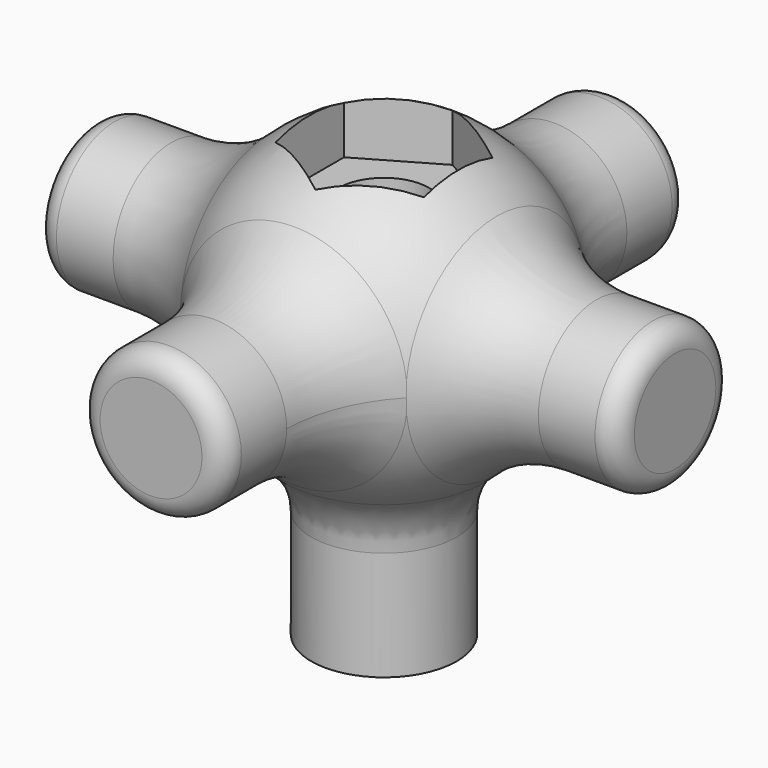
from build123d import *

# Parameters (mm, degrees)
F2_R          = 5
F3_DEPTH      = 20
F4_R          = 5
F5_DEPTH      = 20
F6_R          = 5
F7_DEPTH      = 20
F8_W          = 8.7868496776
F8_H          = 12.2011639178
F9_DEPTH      = 25
F11_DEPTH     = 19
F12_R         = 3.1
F13_DEPTH     = 43.50571
F15_R         = 5
F16_T2_ANGLE  = 180
F16_T4_ANGLE  = 180
F16_T6_ANGLE  = 180
F16_T8_ANGLE  = 180
F16_T10_ANGLE = 179.9999999891
F16_T12_ANGLE = 180.0000000129
F17_R         = 1.5
F18_R         = 1.5


# Not quite as in the source:
# - a fillet or chamfer that OpenCascade refuses, or shapes differently, is made with other operations: its cross-section is extruded or revolved along the edge and cut away or added


with BuildPart() as f1:
    # F0 (on Top) → F1 (revolve)
    with BuildSketch(Plane.XY):
        with BuildLine():
            ThreePointArc((-11, 0), (0, -11), (11, 0))
            Line((11, 0), (-11, 0))
        make_face()
    revolve(axis=Axis((0.2873940393, 0, 0), (1, 0, 0)))

    # F2 (on Top) → F3 (join)
    with BuildSketch(Plane.XY):
        Circle(F2_R)
    extrude(amount=-F3_DEPTH)

    # F4 (on Front) → F5 (join, symmetric)
    with BuildSketch(Plane.XZ):
        Circle(F4_R)
    extrude(amount=F5_DEPTH, both=True)

    # F6 (on Right) → F7 (join, symmetric)
    with BuildSketch(Plane.YZ):
        Circle(F6_R)
    extrude(amount=F7_DEPTH, both=True)

    # F10 (on face) → F11 (cut)
    with BuildSketch(Plane.XY.offset(25)):
        Polygon((-5.1, 2.9444863729), (-5.1, -2.9444863729), (0, -5.8889727457), (5.1, -2.9444863729), (5.1, 2.9444863729), (0, 5.8889727457), align=None)
    extrude(amount=-F11_DEPTH, mode=Mode.SUBTRACT)

    # F12 (on face) → F13 (cut)
    with BuildSketch(Plane.XY.offset(6)):
        Circle(F12_R)
    extrude(amount=-F13_DEPTH, mode=Mode.SUBTRACT)

    # F15
    f15_edges = [f1.edges().sort_by_distance(p)[0] for p in [
        (-5, 0, -9.797959),
    ]]
    fillet(f15_edges, radius=F15_R)

    # F16: fillet of radius 10 on 7 edges, made by hand

    # F16_s1 → F16_t2 (revolve)
    with BuildSketch(Plane.XY):
        with BuildLine():
            ThreePointArc((7.6978109292, -7.8571564232), (10.9173830992, -5.7415035459), (14.6977549306, -4.9996))
            Line((14.6977549306, -4.9996), (14.6977549306, -3.99936))
            ThreePointArc((14.6977549306, -3.99936), (12.2478569509, -3.99976), (9.7979589711, -3.99976))
            Line((9.7979589711, -3.99976), (8.9070216547, -4.5453454545))
            ThreePointArc((8.9070216547, -4.5453454545), (8.0579387192, -5.9215558476), (6.997816529, -7.1426720655))
            Line((6.997816529, -7.1426720655), (7.6978109292, -7.8571564232))
        make_face()
    revolve(axis=Axis((9.7979589711, 0, 0), (1, 0, 0)), revolution_arc=F16_T2_ANGLE)

    # F16_s3 → F16_t4 (revolve)
    with BuildSketch(Plane.XY):
        with BuildLine():
            ThreePointArc((7.6978109292, 7.8571564232), (10.9173830992, 5.7415035459), (14.6977549306, 4.9996))
            Line((14.6977549306, 4.9996), (14.6977549306, 3.99936))
            ThreePointArc((14.6977549306, 3.99936), (12.2478569509, 3.99976), (9.7979589711, 3.99976))
            Line((9.7979589711, 3.99976), (8.9070216547, 4.5453454545))
            ThreePointArc((8.9070216547, 4.5453454545), (8.0579387192, 5.9215558476), (6.997816529, 7.1426720655))
            Line((6.997816529, 7.1426720655), (7.6978109292, 7.8571564232))
        make_face()
    revolve(axis=Axis((9.7979589711, 0, 0), (1, 0, 0)), revolution_arc=F16_T4_ANGLE)

    # F16_s5 → F16_t6 (revolve)
    with BuildSketch(Plane.XY):
        with BuildLine():
            ThreePointArc((-7.6978109292, 7.8571564232), (-10.9173830992, 5.7415035459), (-14.6977549306, 4.9996))
            Line((-14.6977549306, 4.9996), (-14.6977549306, 3.99936))
            ThreePointArc((-14.6977549306, 3.99936), (-12.2478569509, 3.99976), (-9.7979589711, 3.99976))
            Line((-9.7979589711, 3.99976), (-8.9070216547, 4.5453454545))
            ThreePointArc((-8.9070216547, 4.5453454545), (-8.0579387192, 5.9215558476), (-6.997816529, 7.1426720655))
            Line((-6.997816529, 7.1426720655), (-7.6978109292, 7.8571564232))
        make_face()
    revolve(axis=Axis((-9.7979589711, 0, 0), (1, 0, 0)), revolution_arc=F16_T6_ANGLE)

    # F16_s7 → F16_t8 (revolve)
    with BuildSketch(Plane.XY):
        with BuildLine():
            ThreePointArc((-7.6978109292, -7.8571564232), (-10.9173830992, -5.7415035459), (-14.6977549306, -4.9996))
            Line((-14.6977549306, -4.9996), (-14.6977549306, -3.99936))
            ThreePointArc((-14.6977549306, -3.99936), (-12.2478569509, -3.99976), (-9.7979589711, -3.99976))
            Line((-9.7979589711, -3.99976), (-8.9070216547, -4.5453454545))
            ThreePointArc((-8.9070216547, -4.5453454545), (-8.0579387192, -5.9215558476), (-6.997816529, -7.1426720655))
            Line((-6.997816529, -7.1426720655), (-7.6978109292, -7.8571564232))
        make_face()
    revolve(axis=Axis((-9.7979589711, 0, 0), (1, 0, 0)), revolution_arc=F16_T8_ANGLE)

    # F16_s9 → F16_t10 (revolve)
    with BuildSketch(Plane.XY):
        with BuildLine():
            ThreePointArc((7.857156424, -7.6978109292), (5.7415035468, -10.9173830992), (4.9996000008, -14.6977549306))
            Line((4.9996000008, -14.6977549306), (3.9993600008, -14.6977549306))
            ThreePointArc((3.9993600008, -14.6977549306), (3.9997600008, -12.2478569509), (3.99976, -9.7979589711))
            Line((3.99976, -9.7979589711), (4.5453454546, -8.9070216546))
            ThreePointArc((4.5453454546, -8.9070216546), (5.9215558482, -8.0579387193), (7.1426720664, -6.997816529))
            Line((7.1426720664, -6.997816529), (7.857156424, -7.6978109292))
        make_face()
    revolve(axis=Axis((4e-10, -9.7979589711, -5e-10), (0, -1, 0)), revolution_arc=F16_T10_ANGLE)

    # F16_s11 → F16_t12 (revolve)
    with BuildSketch(Plane.XY):
        with BuildLine():
            ThreePointArc((-7.8571564226, -7.6978109292), (-5.7415035453, -10.9173830992), (-4.9995999994, -14.6977549306))
            Line((-4.9995999994, -14.6977549306), (-3.9993599994, -14.6977549306))
            ThreePointArc((-3.9993599994, -14.6977549306), (-3.9997599994, -12.2478569509), (-3.99976, -9.7979589711))
            Line((-3.99976, -9.7979589711), (-4.5453454545, -8.9070216547))
            ThreePointArc((-4.5453454545, -8.9070216547), (-5.9215558472, -8.057938719), (-7.142672065, -6.997816529))
            Line((-7.142672065, -6.997816529), (-7.8571564226, -7.6978109292))
        make_face()
    revolve(axis=Axis((0, -9.7979589711, -6e-10), (0, -1, 0)), revolution_arc=F16_T12_ANGLE)

    # F16_s13 → F16_t14 (revolve)
    with BuildSketch(Plane.XY):
        with BuildLine():
            ThreePointArc((7.8571564244, 7.6978109292), (5.7415035471, 10.9173830992), (4.9996000012, 14.6977549306))
            Line((4.9996000012, 14.6977549306), (3.9993600012, 14.6977549306))
            ThreePointArc((3.9993600012, 14.6977549306), (3.9997600012, 12.2478569509), (3.99976, 9.7979589711))
            Line((3.99976, 9.7979589711), (4.5453454546, 8.9070216546))
            ThreePointArc((4.5453454546, 8.9070216546), (5.9215558484, 8.0579387194), (7.1426720667, 6.997816529))
            Line((7.1426720667, 6.997816529), (7.8571564244, 7.6978109292))
        make_face()
    revolve(axis=Axis((6e-10, 9.7979589711, 1e-10), (0, -1, 0)))

    # F17
    f17_edges = [f1.edges().sort_by_distance(p)[0] for p in [
        (-5, 20, 0),
    ]]
    fillet(f17_edges, radius=F17_R)

    # F18
    f18_edges = [f1.edges().sort_by_distance(p)[0] for p in [
        (20, -5, 0),
        (-5, -20, 0),
        (-20, -5, 0),
    ]]
    fillet(f18_edges, radius=F18_R)


with BuildPart() as f9:
    # F8 (on Top) → F9 (new body)
    with BuildSketch(Plane.XY):
        with Locations((-58.0849088728, 46.795187518)):
            Rectangle(F8_W, F8_H)
    extrude(amount=F9_DEPTH)


solid = f1.part
